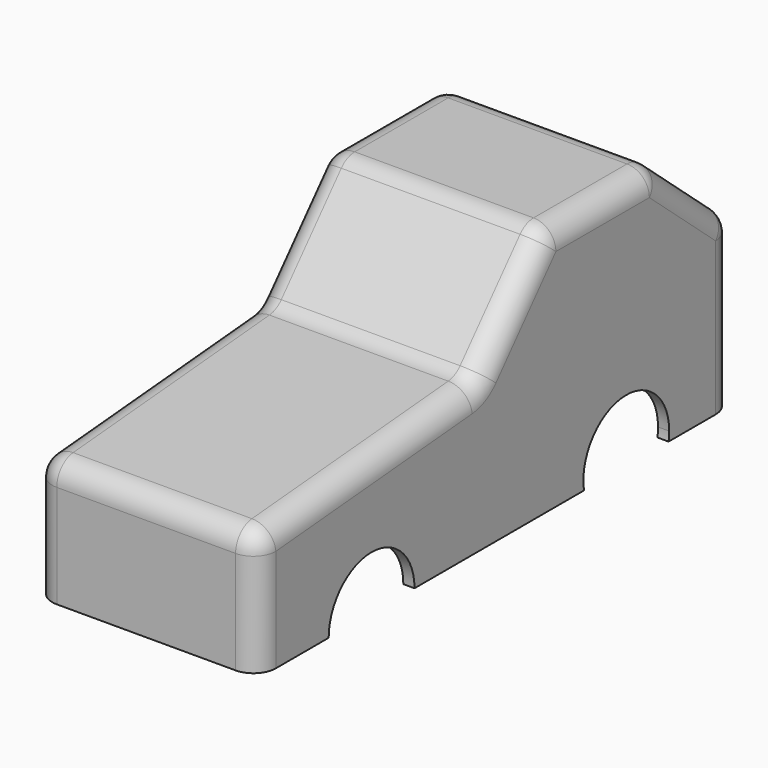
from build123d import *

# Parameters (mm, degrees)
F1_DEPTH = 25
F2_DEPTH = 25
F3_T     = -2.5
F4_R     = 5
F5_DEPTH = 50


with BuildPart() as f1:
    # F0 (on Right) → F1 (new body)
    with BuildSketch(Plane.YZ):
        with BuildLine():
            Line((-61.460785, 27.62407), (-61.460785, 0))
            Line((-61.460785, 0), (-41.680785, 0))
            ThreePointArc((-41.680785, 0), (-29.680785, 12), (-17.680785, 0))
            Line((-17.680785, 0), (29.707056, 0))
            ThreePointArc((29.707056, 0), (40.5357, 13.957966), (53.539215, 2))
            ThreePointArc((53.539215, 2), (53.497181, 0.996485), (53.371375, 0))
            Line((53.371375, 0), (71.539215, 0))
            Line((71.539215, 0), (71.539215, 36.465518))
            Line((71.539215, 36.465518), (49.849141, 55.24814))
            Line((49.849141, 55.24814), (19.590519, 55.24814))
            Line((19.590519, 55.24814), (0, 32.974139))
            Line((0, 32.974139), (-61.460785, 27.62407))
        make_face()
        with BuildLine():
            ThreePointArc((-17.680785, 0), (-29.680785, 12), (-41.680785, 0))
            Line((-41.680785, 0), (-17.680785, 0))
        make_face()
        with BuildLine():
            ThreePointArc((53.539215, 2), (40.5357, 13.957966), (29.707056, 0))
            Line((29.707056, 0), (53.371375, 0))
            ThreePointArc((53.371375, 0), (53.497181, 0.996485), (53.539215, 2))
        make_face()
    extrude(amount=F1_DEPTH)

    # F2 (add): a face of the model
    f2_faces = [f1.faces().sort_by_distance(p)[0] for p in [
        (0, 13.223241, 21.705819),
    ]]
    extrude(f2_faces, amount=F2_DEPTH)

    # F3
    f3_openings = [f1.faces().sort_by_distance(p)[0] for p in [
        (0, 5.039215, 0),
    ]]
    offset(amount=F3_T, openings=f3_openings, kind=Kind.INTERSECTION)

    # F4
    f4_edges = [f1.edges().sort_by_distance(p)[0] for p in [
        (-25, -61.460785, 13.812035),
        (0, -61.460785, 27.62407),
        (25, -61.460785, 13.812035),
        (25, -30.730392, 30.299104),
        (-25, -30.730392, 30.299104),
        (0, 71.539215, 36.465518),
        (25, 34.71983, 55.24814),
        (25, 9.79526, 44.111139),
        (0, 0, 32.974139),
        (-25, 9.79526, 44.111139),
        (0, 19.590519, 55.24814),
        (-25, 34.71983, 55.24814),
        (0, 49.849141, 55.24814),
        (-25, 71.539215, 18.232759),
        (25, 71.539215, 18.232759),
        (25, 60.694178, 45.856829),
        (-25, 60.694178, 45.856829),
    ]]
    fillet(f4_edges, radius=F4_R)

    # F0 (on Right) → F5 (cut, symmetric)
    with BuildSketch(Plane.YZ):
        with BuildLine():
            ThreePointArc((53.539215, 2), (40.5357, 13.957966), (29.707056, 0))
            Line((29.707056, 0), (53.371375, 0))
            ThreePointArc((53.371375, 0), (53.497181, 0.996485), (53.539215, 2))
        make_face()
        with BuildLine():
            ThreePointArc((-17.680785, 0), (-29.680785, 12), (-41.680785, 0))
            Line((-41.680785, 0), (-17.680785, 0))
        make_face()
    extrude(amount=F5_DEPTH, both=True, mode=Mode.SUBTRACT)


solid = f1.part
